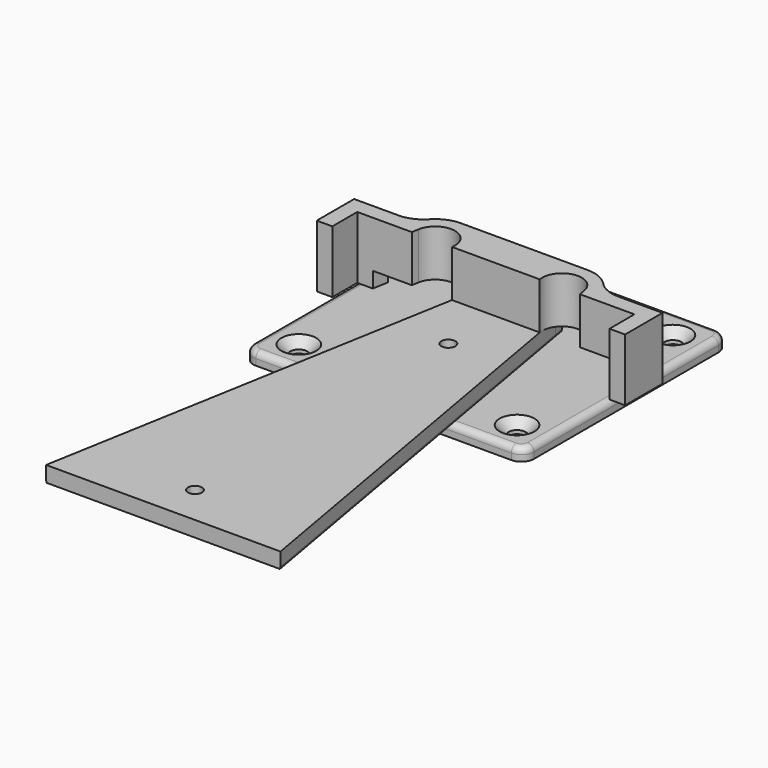
from build123d import *

# Parameters (mm, degrees)
F1_DEPTH       = 4
F2_DEPTH       = 4
F3_T1_DEPTH    = 17.102949117
F3_T3_DEPTH    = 8.5514745585
F3_T5_DEPTH    = 8.5514745585
F3_T8_ANGLE    = 260.0707852325
F3_T10_ANGLE   = 79.9682730154
F4_D           = 5.5
F4_DEPTH       = 8
F4_CSINK_D     = 11.2
F4_CSINK_ANGLE = 90
F4_TIP         = 1.6523667023
F5_R           = 2
F7_DEPTH       = 5
F8_START       = 5
F8_DEPTH       = 15
F9_DEPTH       = 5
F10_D          = 4.4958
F10_DEPTH      = 8
F10_TIP        = 1.3506745855
F11_C1_SIZE2   = 0.2
F11_C1_SIZE    = 0.7
F11_C2_SIZE2   = 0.7
F11_C2_SIZE    = 0.2
F12_R          = 10


# Not quite as in the source:
# - a fillet or chamfer that OpenCascade refuses, or shapes differently, is made with other operations: its cross-section is extruded or revolved along the edge and cut away or added
# - a feature names something its author has since deleted; it is built from what else it names


with BuildPart() as f1:
    # F0 (on Top) → F1 (new body)
    with BuildSketch(Plane.XY):
        with BuildLine():
            Line((-41, -45), (41, -45))
            ThreePointArc((41, -45), (43.8284271247, -43.8284271247), (45, -41))
            Line((45, -41), (45, 33))
            ThreePointArc((45, 33), (43.8284271247, 35.8284271247), (41, 37))
            Line((41, 37), (-41, 37))
            ThreePointArc((-41, 37), (-43.8284271247, 35.8284271247), (-45, 33))
            Line((-45, 33), (-45, -41))
            ThreePointArc((-45, -41), (-43.8284271247, -43.8284271247), (-41, -45))
        make_face()
        with BuildLine():
            Line((-10, -26.8614066163), (-10, -6.6332495807))
            ThreePointArc((-10, -6.6332495807), (0, 12), (10, -6.6332495807))
            Line((10, -6.6332495807), (10, -26.8614066163))
            ThreePointArc((10, -26.8614066163), (0, -30), (-10, -26.8614066163))
        make_face(mode=Mode.SUBTRACT)
        with BuildLine():
            ThreePointArc((-5.2916666667, -3.5100945698), (-1.8330871047, 6.0796621343), (6.35, 0))
            ThreePointArc((6.35, 0), (6.0796621343, -1.8330871047), (5.2916666667, -3.5100945698))
            Line((5.2916666667, -3.5100945698), (10, -6.6332495807))
            ThreePointArc((10, -6.6332495807), (0, 12), (-10, -6.6332495807))
            Line((-10, -6.6332495807), (-5.2916666667, -3.5100945698))
        make_face()
    extrude(amount=-F1_DEPTH)

    # F0 (on Top) → F2 (join)
    with BuildSketch(Plane.XY):
        with BuildLine():
            ThreePointArc((-5.2916666667, -3.5100945698), (-1.8330871047, 6.0796621343), (6.35, 0))
            ThreePointArc((6.35, 0), (6.0796621343, -1.8330871047), (5.2916666667, -3.5100945698))
            Line((5.2916666667, -3.5100945698), (10, -6.6332495807))
            ThreePointArc((10, -6.6332495807), (0, 12), (-10, -6.6332495807))
            Line((-10, -6.6332495807), (-5.2916666667, -3.5100945698))
        make_face()
    extrude(amount=F2_DEPTH)

    # F3: chamfer of 2 on 5 edges, made by hand

    # F3_s2 → F3_t1 (cut)
    with BuildSketch(Plane.XY.offset(-8.5514745585)):
        with BuildLine():
            Line((-5.9783737827, -2.1404548382), (-6.7557845584, -4.481280509))
            Line((-6.7557845584, -4.481280509), (-5.2916666667, -3.5100945698))
            ThreePointArc((-5.2916666667, -3.5100945698), (-5.6892505447, -2.8204482338), (-5.9783737827, -2.1404548382))
        make_face()
    extrude(amount=F3_T1_DEPTH, mode=Mode.SUBTRACT)

    # F3_s4 → F3_t3 (cut)
    with BuildSketch(Plane.XY.offset(-8.5514745585)):
        with BuildLine():
            Line((5.9783737827, -2.1404548382), (6.7557845584, -4.481280509))
            Line((6.7557845584, -4.481280509), (5.2916666667, -3.5100945698))
            ThreePointArc((5.2916666667, -3.5100945698), (5.6892505447, -2.8204482338), (5.9783737827, -2.1404548382))
        make_face()
    extrude(amount=F3_T3_DEPTH, mode=Mode.SUBTRACT)

    # F3_s6 → F3_t5 (cut)
    with BuildSketch(Plane.XY):
        with BuildLine():
            Line((5.9783737827, -2.1404548382), (6.7557845584, -4.481280509))
            Line((6.7557845584, -4.481280509), (5.2916666667, -3.5100945698))
            ThreePointArc((5.2916666667, -3.5100945698), (5.6892505447, -2.8204482338), (5.9783737827, -2.1404548382))
        make_face()
    extrude(amount=F3_T5_DEPTH, mode=Mode.SUBTRACT)

    # F3_s7 → F3_t8 (revolve, cut)
    with BuildSketch(Plane(origin=(0, 0, 0), x_dir=(0, 0, 1), z_dir=(0.9850215325, -0.1724313791, 0))):
        Polygon((2, 6.35), (4, 8.35), (4, 6.35), align=None)
    revolve(axis=Axis((0, 0, 4), (0, 0, -1)), revolution_arc=F3_T8_ANGLE, mode=Mode.SUBTRACT)

    # F3_s9 → F3_t10 (revolve, cut)
    with BuildSketch(Plane.XZ):
        Polygon((8.35, 4), (6.35, 2), (6.35, 4), align=None)
    revolve(axis=Axis((0, 0, 4), (0, 0, -1)), revolution_arc=F3_T10_ANGLE, mode=Mode.SUBTRACT)

    # F4
    with Locations(Plane.XY):
        with Locations((-35, 27.25), (-35, -35.25), (35, -35.25), (35, 27.25)):
            CounterSinkHole(F4_D / 2, F4_CSINK_D / 2, depth=F4_DEPTH, counter_sink_angle=F4_CSINK_ANGLE)
            with Locations((0, 0, -(F4_DEPTH + F4_TIP / 2))):  # 118° drill point
                Cone(0, F4_D / 2, F4_TIP, mode=Mode.SUBTRACT)

    # F5
    f5_edges = [f1.edges().sort_by_distance(p)[0] for p in [
        (0, -45, 0),
        (-43.828427, -43.828427, 0),
        (43.828427, -43.828427, 0),
        (-43.828427, 35.828427, 0),
        (43.828427, 35.828427, 0),
        (0, 37, 0),
    ]]
    fillet(f5_edges, radius=F5_R)

    # F6 (on Top) → F9 (cut)
    with BuildSketch(Plane.XY):
        with BuildLine():
            Line((12.6607118812, 8.0489585372), (14.0799604379, 0))
            ThreePointArc((14.0799604379, 0), (19.2308237413, 7.3561951598), (26.5870189011, 2.2053318564))
            Line((26.5870189011, 2.2053318564), (26.9758784088, 0))
            Line((26.9758784088, 0), (39.4656266949, 0))
            Line((39.4656266949, 0), (38.5839917914, 5))
            Line((38.5839917914, 5), (29.9216744368, 5))
            ThreePointArc((29.9216744368, 5), (26.1121180689, 9.6892807339), (20.3334896695, 11.4526659282))
            ThreePointArc((20.3334896695, 11.4526659282), (16.1365639198, 10.5635493041), (12.6607118812, 8.0489585372))
        make_face()
        with BuildLine():
            ThreePointArc((-26.5870189011, 2.2053318564), (-19.2308237413, 7.3561951598), (-14.0799604379, 0))
            Line((-14.0799604379, 0), (-12.6607118812, 8.0489585372))
            ThreePointArc((-12.6607118812, 8.0489585372), (-16.1365639198, 10.5635493041), (-20.3334896695, 11.4526659282))
            ThreePointArc((-20.3334896695, 11.4526659282), (-26.1121180689, 9.6892807339), (-29.9216744368, 5))
            Line((-29.9216744368, 5), (-38.5839908315, 5))
            Line((-38.5839908315, 5), (-39.465625735, 0))
            Line((-39.465625735, 0), (-26.9758784088, 0))
            Line((-26.9758784088, 0), (-26.5870189011, 2.2053318564))
        make_face()
    extrude(amount=F9_DEPTH, mode=Mode.SUBTRACT)


with BuildPart() as f7:
    # F6 (on Top) → F7 (new body)
    with BuildSketch(Plane.XY):
        Polygon((-14.0799604379, 0), (-37.5931633153, -133.35), (37.5931633153, -133.35), (14.0799604379, 0), align=None)
        with BuildLine():
            Line((-12.6607118812, 8.0489585372), (-14.0799604379, 0))
            Line((-14.0799604379, 0), (14.0799604379, 0))
            Line((14.0799604379, 0), (12.6607118812, 8.0489585372))
            ThreePointArc((12.6607118812, 8.0489585372), (11.5694013468, 6.6084134589), (10.7453049022, 5))
            Line((10.7453049022, 5), (-10.7453049022, 5))
            ThreePointArc((-10.7453049022, 5), (-11.5694013468, 6.6084134589), (-12.6607118812, 8.0489585372))
        make_face()
        with BuildLine():
            Line((-12.0605464337, 11.4526659282), (-12.6607118812, 8.0489585372))
            ThreePointArc((-12.6607118812, 8.0489585372), (-11.5694013468, 6.6084134589), (-10.7453049022, 5))
            Line((-10.7453049022, 5), (10.7453049022, 5))
            ThreePointArc((10.7453049022, 5), (11.5694013468, 6.6084134589), (12.6607118812, 8.0489585372))
            Line((12.6607118812, 8.0489585372), (12.0605464337, 11.4526659282))
            Line((12.0605464337, 11.4526659282), (-12.0605464337, 11.4526659282))
        make_face()
    extrude(amount=F7_DEPTH)



with BuildPart() as f7b:
    # F6 (on Top) → F7, piece 2 (new body)
    with BuildSketch(Plane.XY):
        Polygon((38.5839917914, 5), (39.4656266949, 0), (44.45, 0), (44.45, -10), (49.45, -10), (49.45, 5), align=None)
    extrude(amount=F7_DEPTH)


with BuildPart() as f7c:
    # F6 (on Top) → F7, piece 3 (new body)
    with BuildSketch(Plane.XY):
        Polygon((-44.45, 0), (-39.465625735, 0), (-38.5839908315, 5), (-49.45, 5), (-49.45, -10), (-44.45, -10), align=None)
    extrude(amount=F7_DEPTH)


with BuildPart() as f7_1:
    add(f7.part)

    add(f7b.part)  # F8 merges F7b

    add(f7c.part)  # F8 merges F7c
    # F6 (on Top) → F8 (join)
    with BuildSketch(Plane.XY.offset(F8_START)):
        with BuildLine():
            Line((12.6607118812, 8.0489585372), (14.0799604379, 0))
            ThreePointArc((14.0799604379, 0), (19.2308237413, 7.3561951598), (26.5870189011, 2.2053318564))
            Line((26.5870189011, 2.2053318564), (26.9758784088, 0))
            Line((26.9758784088, 0), (39.4656266949, 0))
            Line((39.4656266949, 0), (38.5839917914, 5))
            Line((38.5839917914, 5), (29.9216744368, 5))
            ThreePointArc((29.9216744368, 5), (26.1121180689, 9.6892807339), (20.3334896695, 11.4526659282))
            ThreePointArc((20.3334896695, 11.4526659282), (16.1365639198, 10.5635493041), (12.6607118812, 8.0489585372))
        make_face()
        Polygon((38.5839917914, 5), (39.4656266949, 0), (44.45, 0), (44.45, -10), (49.45, -10), (49.45, 5), align=None)
        with BuildLine():
            ThreePointArc((-26.5870189011, 2.2053318564), (-19.2308237413, 7.3561951598), (-14.0799604379, 0))
            Line((-14.0799604379, 0), (-12.6607118812, 8.0489585372))
            ThreePointArc((-12.6607118812, 8.0489585372), (-16.1365639198, 10.5635493041), (-20.3334896695, 11.4526659282))
            ThreePointArc((-20.3334896695, 11.4526659282), (-26.1121180689, 9.6892807339), (-29.9216744368, 5))
            Line((-29.9216744368, 5), (-38.5839908315, 5))
            Line((-38.5839908315, 5), (-39.465625735, 0))
            Line((-39.465625735, 0), (-26.9758784088, 0))
            Line((-26.9758784088, 0), (-26.5870189011, 2.2053318564))
        make_face()
        Polygon((-44.45, 0), (-39.465625735, 0), (-38.5839908315, 5), (-49.45, 5), (-49.45, -10), (-44.45, -10), align=None)
        with BuildLine():
            Line((-12.6607118812, 8.0489585372), (-14.0799604379, 0))
            Line((-14.0799604379, 0), (14.0799604379, 0))
            Line((14.0799604379, 0), (12.6607118812, 8.0489585372))
            ThreePointArc((12.6607118812, 8.0489585372), (11.5694013468, 6.6084134589), (10.7453049022, 5))
            Line((10.7453049022, 5), (-10.7453049022, 5))
            ThreePointArc((-10.7453049022, 5), (-11.5694013468, 6.6084134589), (-12.6607118812, 8.0489585372))
        make_face()
        with BuildLine():
            Line((-12.0605464337, 11.4526659282), (-12.6607118812, 8.0489585372))
            ThreePointArc((-12.6607118812, 8.0489585372), (-11.5694013468, 6.6084134589), (-10.7453049022, 5))
            Line((-10.7453049022, 5), (10.7453049022, 5))
            ThreePointArc((10.7453049022, 5), (11.5694013468, 6.6084134589), (12.6607118812, 8.0489585372))
            Line((12.6607118812, 8.0489585372), (12.0605464337, 11.4526659282))
            Line((12.0605464337, 11.4526659282), (-12.0605464337, 11.4526659282))
        make_face()
        with BuildLine():
            Line((12.0605464337, 11.4526659282), (12.6607118812, 8.0489585372))
            ThreePointArc((12.6607118812, 8.0489585372), (16.1365639198, 10.5635493041), (20.3334896695, 11.4526659282))
            Line((20.3334896695, 11.4526659282), (12.0605464337, 11.4526659282))
        make_face()
        with BuildLine():
            ThreePointArc((-20.3334896695, 11.4526659282), (-16.1365639198, 10.5635493041), (-12.6607118812, 8.0489585372))
            Line((-12.6607118812, 8.0489585372), (-12.0605464337, 11.4526659282))
            Line((-12.0605464337, 11.4526659282), (-20.3334896695, 11.4526659282))
        make_face()
    extrude(amount=F8_DEPTH)

    # F10
    with Locations(Plane(origin=(0, 0, 0), x_dir=(1, 0, 0), z_dir=(0, 0, -1))):
        with Locations((0, 19.05), (0, 120.65)):
            Hole(F10_D / 2, depth=F10_DEPTH)
            with Locations((0, 0, -(F10_DEPTH + F10_TIP / 2))):  # 118° drill point
                Cone(0, F10_D / 2, F10_TIP, mode=Mode.SUBTRACT)

    # F11: chamfer of 0.2 x 0.7 on 2 edges, made by hand

    # F11_c1
    f11_c1_edges = [f7_1.edges().sort_by_distance(p)[0] for p in [
        (-24.8268548745, -60.9486670359, 0),
    ]]
    f11_c1_side = f7_1.faces().sort_by_distance((-24.8268548745, -60.9486670359, 0.004))[0]
    chamfer(f11_c1_edges, length=F11_C1_SIZE, length2=F11_C1_SIZE2, reference=f11_c1_side)

    # F11_c2
    f11_c2_edges = [f7_1.edges().sort_by_distance(p)[0] for p in [
        (24.8268548745, -60.9486670359, 0),
    ]]
    f11_c2_side = f7_1.faces().sort_by_distance((24.8229156435, -60.9493616286, 0))[0]
    chamfer(f11_c2_edges, length=F11_C2_SIZE, length2=F11_C2_SIZE2, reference=f11_c2_side)

    # F12
    f12_edges = [f7_1.edges().sort_by_distance(p)[0] for p in [
        (29.921674, 5, 12.5),
        (-29.921674, 5, 12.5),
    ]]
    fillet(f12_edges, radius=F12_R)


solid = Compound([f1.part, f7_1.part])
